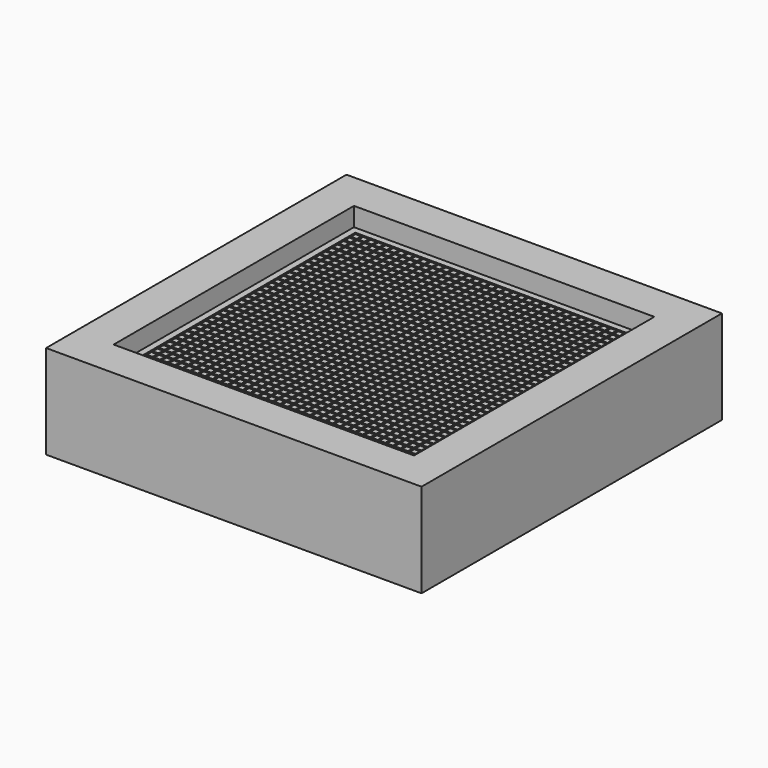
from build123d import *

# Parameters (mm, degrees)
F0_W     = 100
F0_H     = 100
F1_DEPTH = 25
F2_W     = 80
F2_H     = 80
F3_DEPTH = 5
F4_W     = 0.5
F4_H     = 76.5
F5_DEPTH = 0.2
F6_W     = 76
F6_H     = 0.5
F7_DEPTH = 0.2


with BuildPart() as f1:
    # F0 (on Top) → F1 (new body)
    with BuildSketch(Plane.XY):
        with Locations((50, 50)):
            Rectangle(F0_W, F0_H)
    extrude(amount=F1_DEPTH)

    # F2 (on face) → F3 (cut)
    with BuildSketch(Plane.XY.offset(25)):
        with Locations((50, 50)):
            Rectangle(F2_W, F2_H)
    extrude(amount=-F3_DEPTH, mode=Mode.SUBTRACT)

    # F4 (on face) → F5 (cut)
    with BuildSketch(Plane.XY.offset(20)):
        with Locations((12, 50)):
            Rectangle(F4_W, F4_H)
        with Locations((14, 50)):
            Rectangle(F4_W, F4_H)
        with Locations((16, 50)):
            Rectangle(F4_W, F4_H)
        with Locations((18, 50)):
            Rectangle(F4_W, F4_H)
        with Locations((20, 50)):
            Rectangle(F4_W, F4_H)
        with Locations((22, 50)):
            Rectangle(F4_W, F4_H)
        with Locations((24, 50)):
            Rectangle(F4_W, F4_H)
        with Locations((26, 50)):
            Rectangle(F4_W, F4_H)
        with Locations((28, 50)):
            Rectangle(F4_W, F4_H)
        with Locations((30, 50)):
            Rectangle(F4_W, F4_H)
        with Locations((32, 50)):
            Rectangle(F4_W, F4_H)
        with Locations((34, 50)):
            Rectangle(F4_W, F4_H)
        with Locations((36, 50)):
            Rectangle(F4_W, F4_H)
        with Locations((38, 50)):
            Rectangle(F4_W, F4_H)
        with Locations((40, 50)):
            Rectangle(F4_W, F4_H)
        with Locations((42, 50)):
            Rectangle(F4_W, F4_H)
        with Locations((44, 50)):
            Rectangle(F4_W, F4_H)
        with Locations((46, 50)):
            Rectangle(F4_W, F4_H)
        with Locations((48, 50)):
            Rectangle(F4_W, F4_H)
        with Locations((50, 50)):
            Rectangle(F4_W, F4_H)
        with Locations((52, 50)):
            Rectangle(F4_W, F4_H)
        with Locations((54, 50)):
            Rectangle(F4_W, F4_H)
        with Locations((56, 50)):
            Rectangle(F4_W, F4_H)
        with Locations((58, 50)):
            Rectangle(F4_W, F4_H)
        with Locations((60, 50)):
            Rectangle(F4_W, F4_H)
        with Locations((62, 50)):
            Rectangle(F4_W, F4_H)
        with Locations((64, 50)):
            Rectangle(F4_W, F4_H)
        with Locations((66, 50)):
            Rectangle(F4_W, F4_H)
        with Locations((68, 50)):
            Rectangle(F4_W, F4_H)
        with Locations((70, 50)):
            Rectangle(F4_W, F4_H)
        with Locations((72, 50)):
            Rectangle(F4_W, F4_H)
        with Locations((74, 50)):
            Rectangle(F4_W, F4_H)
        with Locations((76, 50)):
            Rectangle(F4_W, F4_H)
        with Locations((78, 50)):
            Rectangle(F4_W, F4_H)
        with Locations((80, 50)):
            Rectangle(F4_W, F4_H)
        with Locations((82, 50)):
            Rectangle(F4_W, F4_H)
        with Locations((84, 50)):
            Rectangle(F4_W, F4_H)
        with Locations((86, 50)):
            Rectangle(F4_W, F4_H)
        with Locations((88, 50)):
            Rectangle(F4_W, F4_H)
    extrude(amount=-F5_DEPTH, mode=Mode.SUBTRACT)

    # F6 (on face) → F7 (cut)
    with BuildSketch(Plane.XY.offset(20)):
        with Locations((50, 88)):
            Rectangle(F6_W, F6_H)
        with Locations((50, 86)):
            Rectangle(F6_W, F6_H)
        with Locations((50, 84)):
            Rectangle(F6_W, F6_H)
        with Locations((50, 82)):
            Rectangle(F6_W, F6_H)
        with Locations((50, 80)):
            Rectangle(F6_W, F6_H)
        with Locations((50, 78)):
            Rectangle(F6_W, F6_H)
        with Locations((50, 76)):
            Rectangle(F6_W, F6_H)
        with Locations((50, 74)):
            Rectangle(F6_W, F6_H)
        with Locations((50, 72)):
            Rectangle(F6_W, F6_H)
        with Locations((50, 70)):
            Rectangle(F6_W, F6_H)
        with Locations((50, 68)):
            Rectangle(F6_W, F6_H)
        with Locations((50, 66)):
            Rectangle(F6_W, F6_H)
        with Locations((50, 64)):
            Rectangle(F6_W, F6_H)
        with Locations((50, 62)):
            Rectangle(F6_W, F6_H)
        with Locations((50, 60)):
            Rectangle(F6_W, F6_H)
        with Locations((50, 58)):
            Rectangle(F6_W, F6_H)
        with Locations((50, 56)):
            Rectangle(F6_W, F6_H)
        with Locations((50, 54)):
            Rectangle(F6_W, F6_H)
        with Locations((50, 52)):
            Rectangle(F6_W, F6_H)
        with Locations((50, 50)):
            Rectangle(F6_W, F6_H)
        with Locations((50, 48)):
            Rectangle(F6_W, F6_H)
        with Locations((50, 46)):
            Rectangle(F6_W, F6_H)
        with Locations((50, 44)):
            Rectangle(F6_W, F6_H)
        with Locations((50, 42)):
            Rectangle(F6_W, F6_H)
        with Locations((50, 40)):
            Rectangle(F6_W, F6_H)
        with Locations((50, 38)):
            Rectangle(F6_W, F6_H)
        with Locations((50, 36)):
            Rectangle(F6_W, F6_H)
        with Locations((50, 34)):
            Rectangle(F6_W, F6_H)
        with Locations((50, 32)):
            Rectangle(F6_W, F6_H)
        with Locations((50, 30)):
            Rectangle(F6_W, F6_H)
        with Locations((50, 28)):
            Rectangle(F6_W, F6_H)
        with Locations((50, 26)):
            Rectangle(F6_W, F6_H)
        with Locations((50, 24)):
            Rectangle(F6_W, F6_H)
        with Locations((50, 22)):
            Rectangle(F6_W, F6_H)
        with Locations((50, 20)):
            Rectangle(F6_W, F6_H)
        with Locations((50, 18)):
            Rectangle(F6_W, F6_H)
        with Locations((50, 16)):
            Rectangle(F6_W, F6_H)
        with Locations((50, 14)):
            Rectangle(F6_W, F6_H)
        with Locations((50, 12)):
            Rectangle(F6_W, F6_H)
    extrude(amount=-F7_DEPTH, mode=Mode.SUBTRACT)


solid = f1.part
